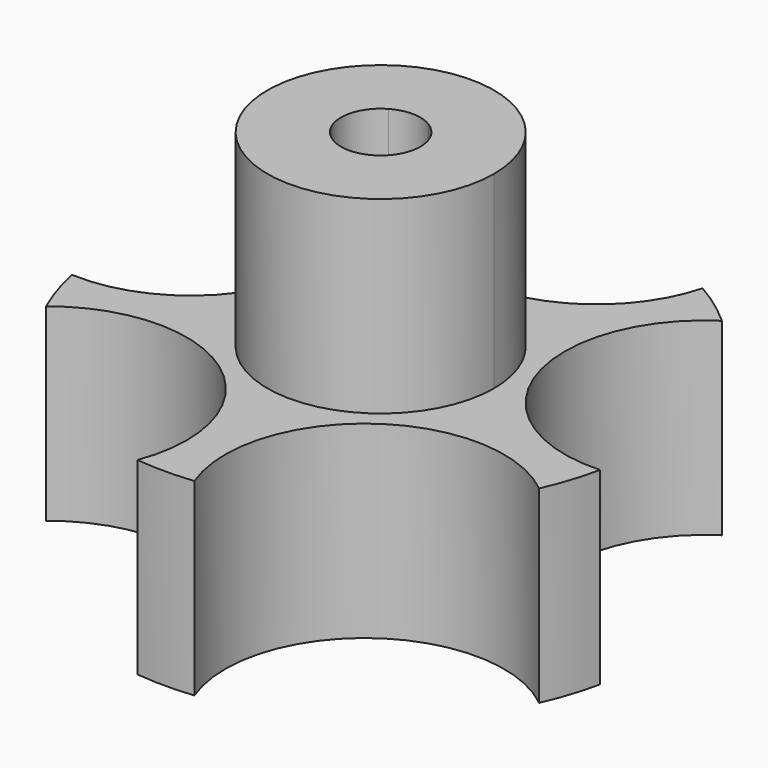
from build123d import *

# Parameters (mm, degrees)
F1_DEPTH = 5
F2_DEPTH = 10
F3_DEPTH = 3


with BuildPart() as f1:
    # F0 (on Top) → F1 (new body)
    with BuildSketch(Plane.XY):
        with BuildLine():
            Line((0.560707187, 3.4989949035), (0.560707187, 2.9471354652))
            ThreePointArc((0.560707187, 2.9471354652), (2.3110735126, 1.9128353874), (3, 0))
            ThreePointArc((3, 0), (-1.9287498107, -2.2978085577), (-0.5199494453, 2.9545985471))
            Line((-0.5199494453, 2.9545985471), (-0.5199494453, 3.4929679604))
            ThreePointArc((-0.5199494453, 3.4929679604), (-2.4505424978, 4.3861128404), (-3.5684511747, 6.1958579885))
            ThreePointArc((-3.5684511747, 6.1958579885), (-4.2026645539, 5.7844715098), (-4.7898990575, 5.3084241559))
            ThreePointArc((-4.7898990575, 5.3084241559), (-3.5543368281, 3.9728631878), (-3.1062443016, 2.2094715098))
            ThreePointArc((-3.1062443016, 2.2094715098), (-4.2581115343, -0.4705954297), (-6.9953231706, -1.4791733296))
            ThreePointArc((-6.9953231706, -1.4791733296), (-6.8000540915, -2.2094715098), (-6.5287715949, -2.9150714334))
            ThreePointArc((-6.5287715949, -2.9150714334), (-2.6133197512, -2.450072934), (-0.508854764, -5.7844715098))
            ThreePointArc((-0.508854764, -5.7844715098), (-0.5708860042, -6.4585748626), (-0.754896307, -7.1100373814))
            ThreePointArc((-0.754896307, -7.1100373814), (0, -7.15), (0.754896307, -7.1100373814))
            ThreePointArc((0.754896307, -7.1100373814), (2.0314976346, -2.7961166157), (6.5287715949, -2.9150714334))
            ThreePointArc((6.5287715949, -2.9150714334), (6.8000540915, -2.2094715098), (6.9953231706, -1.4791733296))
            ThreePointArc((6.9953231706, -1.4791733296), (3.2870322209, 1.0680215107), (4.7898990575, 5.3084241559))
            ThreePointArc((4.7898990575, 5.3084241559), (4.2026645539, 5.7844715098), (3.5684511747, 6.1958579885))
            ThreePointArc((3.5684511747, 6.1958579885), (2.4659186562, 4.3998225611), (0.560707187, 3.4989949035))
        make_face()
        with BuildLine():
            ThreePointArc((-0.5199494453, 2.9545985471), (0.0207176923, 2.999928462), (0.560707187, 2.9471354652))
            Line((0.560707187, 2.9471354652), (0.560707187, 3.4989949035))
            ThreePointArc((0.560707187, 3.4989949035), (0.0206004706, 3.4562476552), (-0.5199494453, 3.4929679604))
            Line((-0.5199494453, 3.4929679604), (-0.5199494453, 2.9545985471))
        make_face()
    extrude(amount=F1_DEPTH)

    # F0 (on Top) → F2 (join)
    with BuildSketch(Plane.XY):
        with BuildLine():
            ThreePointArc((0.560707187, 0.887754161), (0.9195766815, 0.5068320499), (1.05, 0))
            ThreePointArc((1.05, 0), (-0.527519233, -0.9078675337), (-0.5199494453, 0.9122239716))
            Line((-0.5199494453, 0.9122239716), (-0.5199494453, 2.9545985471))
            ThreePointArc((-0.5199494453, 2.9545985471), (-1.9287498107, -2.2978085577), (3, 0))
            ThreePointArc((3, 0), (2.3110735126, 1.9128353874), (0.560707187, 2.9471354652))
            Line((0.560707187, 2.9471354652), (0.560707187, 0.887754161))
        make_face()
        with BuildLine():
            ThreePointArc((-0.5199494453, 0.9122239716), (0.0237695453, 1.0497309221), (0.560707187, 0.887754161))
            Line((0.560707187, 0.887754161), (0.560707187, 2.9471354652))
            ThreePointArc((0.560707187, 2.9471354652), (0.0207176923, 2.999928462), (-0.5199494453, 2.9545985471))
            Line((-0.5199494453, 2.9545985471), (-0.5199494453, 0.9122239716))
        make_face()
    extrude(amount=F2_DEPTH)

    # F0 (on Top) → F3 (cut)
    with BuildSketch(Plane.XY):
        with BuildLine():
            ThreePointArc((-0.5199494453, 0.9122239716), (0.0237695453, 1.0497309221), (0.560707187, 0.887754161))
            Line((0.560707187, 0.887754161), (0.560707187, 2.9471354652))
            ThreePointArc((0.560707187, 2.9471354652), (0.0207176923, 2.999928462), (-0.5199494453, 2.9545985471))
            Line((-0.5199494453, 2.9545985471), (-0.5199494453, 0.9122239716))
        make_face()
        with BuildLine():
            ThreePointArc((-0.5199494453, 2.9545985471), (0.0207176923, 2.999928462), (0.560707187, 2.9471354652))
            Line((0.560707187, 2.9471354652), (0.560707187, 3.4989949035))
            ThreePointArc((0.560707187, 3.4989949035), (0.0206004706, 3.4562476552), (-0.5199494453, 3.4929679604))
            Line((-0.5199494453, 3.4929679604), (-0.5199494453, 2.9545985471))
        make_face()
    extrude(amount=F3_DEPTH, mode=Mode.SUBTRACT)


solid = f1.part
